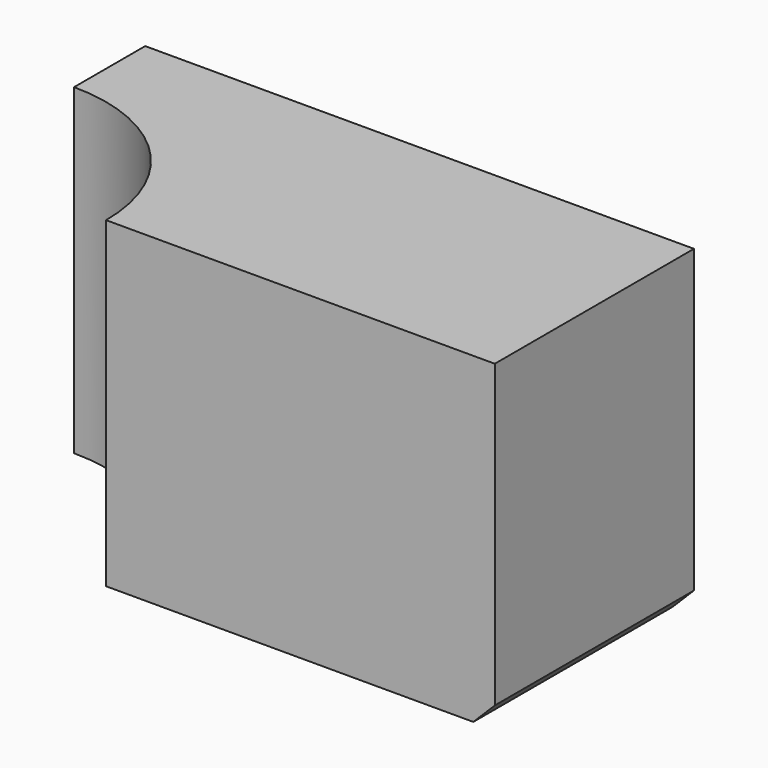
from build123d import *

# Parameters (mm, degrees)
F1_DEPTH = 76.2
F3_SIZE  = 5.08


# Not quite as in the source:
# - the program builds the solid bodies; features that only make, move or delete a surface that nothing else refers to are left out


with BuildPart() as f1:
    # F0 (on Top) → F1 (new body)
    with BuildSketch(Plane.XY):
        with BuildLine():
            ThreePointArc((0, 37.8345108272), (26.7530391688, 26.7530391688), (37.8345108272, 0))
            Line((37.8345108272, 0), (129.7342181206, 0))
            Line((129.7342181206, 0), (129.7342181206, 58.8485188782))
            Line((129.7342181206, 58.8485188782), (0, 58.8485188782))
            Line((0, 58.8485188782), (0, 37.8345108272))
        make_face()
    extrude(amount=F1_DEPTH)

    # F3
    f3_edges = [f1.edges().sort_by_distance(p)[0] for p in [
        (129.734218, 29.424259, 0),
    ]]
    chamfer(f3_edges, length=F3_SIZE)


solid = f1.part
